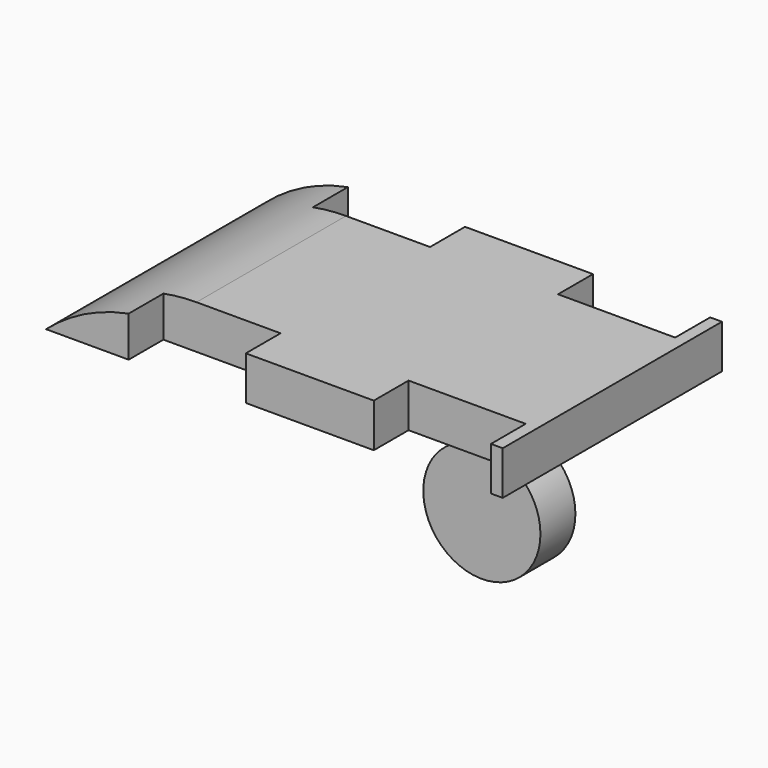
from build123d import *

# Parameters (mm, degrees)
F1_DEPTH    = 12.7
F2_T1_DEPTH = 247.6009079887
F3_R        = 17.0185577346
F4_DEPTH    = 12.7


# Not quite as in the source:
# - a fillet or chamfer that OpenCascade refuses, or shapes differently, is made with other operations: its cross-section is extruded or revolved along the edge and cut away or added


with BuildPart() as f1:
    # F0 (on Top) → F1 (new body)
    with BuildSketch(Plane.XY):
        Polygon((-34.0371176, 31.6446077985), (-58.0253747608, 31.6446077985), (-58.0253747608, -47.9510919376), (-34.0371176, -47.9510919376), (-34.0371176, -35.3372873902), (0, -35.3372873902), (0, -47.9510919376), (37.1790196625, -47.9510919376), (37.1790196625, -35.3372873902), (71.2161372625, -35.3372873902), (71.2161372625, -47.9510919376), (74.6341247993, -47.9510919376), (74.6341247993, 31.6446077985), (71.2161372625, 31.6446077985), (71.2161372625, 18.9446077985), (37.1790196625, 18.9446077985), (37.1790196625, 31.6446077985), (0, 31.6446077985), (0, 18.9446077985), (-34.0371176, 18.9446077985), align=None)
    extrude(amount=F1_DEPTH)

    # F2: fillet of radius 50.8 on 1 edges, made by hand

    # F2_s2 → F2_t1 (cut)
    with BuildSketch(Plane.XZ.offset(-115.6472119248)):
        with BuildLine():
            ThreePointArc((-58.0253747608, 0), (-42.3848453524, 9.419048812), (-24.4243331103, 12.7))
            Line((-24.4243331103, 12.7), (-58.0253747608, 12.7))
            Line((-58.0253747608, 12.7), (-58.0253747608, 0))
        make_face()
    extrude(amount=F2_T1_DEPTH, mode=Mode.SUBTRACT)


with BuildPart() as f4:
    # F3 (on Front) → F4 (new body)
    with BuildSketch(Plane.XZ):
        with Locations((40.3680205345, -29.1869509965)):
            Circle(F3_R)
    extrude(amount=F4_DEPTH)


solid = Compound([f1.part, f4.part])
